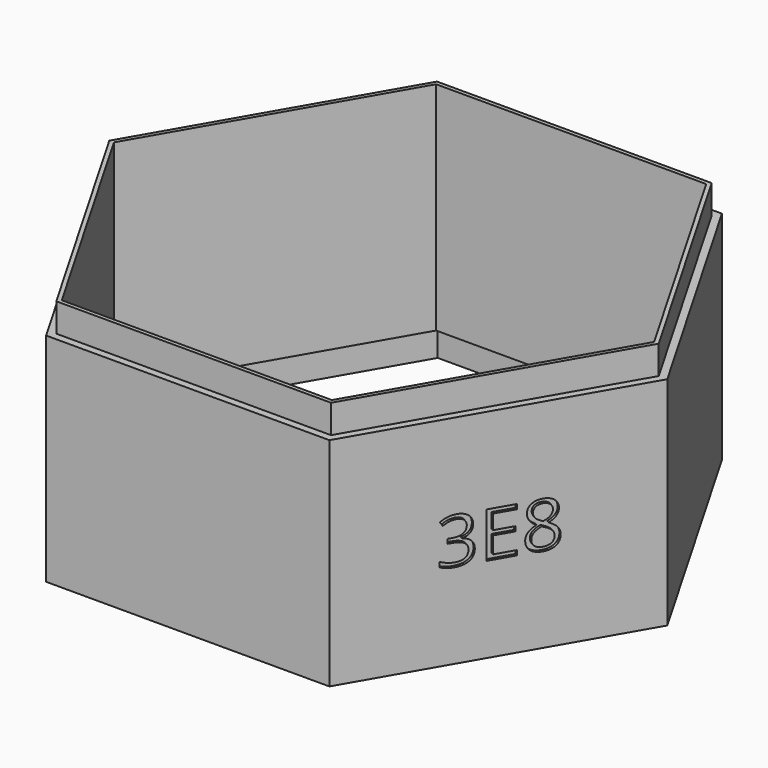
from build123d import *

# Parameters (mm, degrees)
F1_DEPTH      = 2
F3_DEPTH      = 41
F5_DEPTH      = 5
F6_TEXT_SIZE  = 11.1241695575
F7_DEPTH      = 0.5
F8_DEPTH      = 2.0010001
F10_DEPTH     = 5
F11_TEXT_SIZE = 8.3333333333
F12_DEPTH     = 0.5


# Not quite as in the source:
# - Text() gives the source's letters only with a copy of the font that has no kerning and outlines rounded to 1/6400 em; it was checked with that copy


with BuildPart() as f1:
    # F0 (on Top) → F1 (new body)
    with BuildSketch(Plane.XY):
        Polygon((-24.8260615752, -43), (24.8260615752, -43), (49.6521231503, 0), (24.8260615752, 43), (-24.8260615752, 43), (-49.6521231503, 0), align=None)
    extrude(amount=F1_DEPTH)

    # F2 (on face) → F3 (join)
    with BuildSketch(Plane.XY.offset(2)):
        Polygon((-49.6521231503, 0), (-24.8260615752, -43), (24.8260615752, -43), (49.6521231503, 0), (24.8260615752, 43), (-24.8260615752, 43), align=None)
        Polygon((-23.6713610368, 41), (23.6713610368, 41), (47.3427220735, 0), (23.6713610368, -41), (-23.6713610368, -41), (-47.3427220735, 0), align=None, mode=Mode.SUBTRACT)
    extrude(amount=F3_DEPTH)

    # F4 (on face) → F5 (cut)
    with BuildSketch(Plane.XY.offset(43)):
        Polygon((-24.8260615752, 43), (-49.6521231503, 0), (-24.8260615752, -43), (24.8260615752, -43), (49.6521231503, 0), (24.8260615752, 43), align=None)
        Polygon((-24.0755062252, -41.7), (-48.1510124504, 0), (-24.0755062252, 41.7), (24.0755062252, 41.7), (48.1510124504, 0), (24.0755062252, -41.7), align=None, mode=Mode.SUBTRACT)
    extrude(amount=-F5_DEPTH, mode=Mode.SUBTRACT)

    # F6 (on face) → F7 (cut)
    with BuildSketch(Plane(origin=(37.2390923627, -21.5, 0), x_dir=(0.5, 0.8660254038, 0), z_dir=(0.8660254038, -0.5, 0))):
        with Locations((-9.1652728245, 14.9952989593)):
            Text('3E8', F6_TEXT_SIZE, font='Open Sans', text_align=(TextAlign.LEFT, TextAlign.BOTTOM))
    extrude(amount=-F7_DEPTH, mode=Mode.SUBTRACT)

    # F8 (cut, through all): a face of the model
    f8_faces = [f1.faces().sort_by_distance(p)[0] for p in [
        (0, 0, 2),
    ]]
    extrude(f8_faces, amount=-F8_DEPTH, mode=Mode.SUBTRACT)

    # F9 (on face) → F10 (cut)
    with BuildSketch(Plane(origin=(0, 0, 0), x_dir=(1, 0, 0), z_dir=(0, 0, -1))):
        Polygon((24.4219163867, 42.3), (-24.4219163867, 42.3), (-48.8438327734, 0), (-24.4219163867, -42.3), (24.4219163867, -42.3), (48.8438327734, 0), align=None)
        Polygon((-23.6713610368, 41), (23.6713610368, 41), (47.3427220735, 0), (23.6713610368, -41), (-23.6713610368, -41), (-47.3427220735, 0), align=None, mode=Mode.SUBTRACT)
    extrude(amount=-F10_DEPTH, mode=Mode.SUBTRACT)

    # F11 (on face) → F12 (cut)
    with BuildSketch(Plane(origin=(-37.2390923627, -21.5, 0), x_dir=(0.5, -0.8660254038, 0), z_dir=(-0.8660254038, -0.5, 0))):
        with Locations((-18.2076822917, 16)):
            Text('Seafarers', F11_TEXT_SIZE, font='Open Sans', text_align=(TextAlign.LEFT, TextAlign.BOTTOM))
    extrude(amount=-F12_DEPTH, mode=Mode.SUBTRACT)


solid = f1.part
